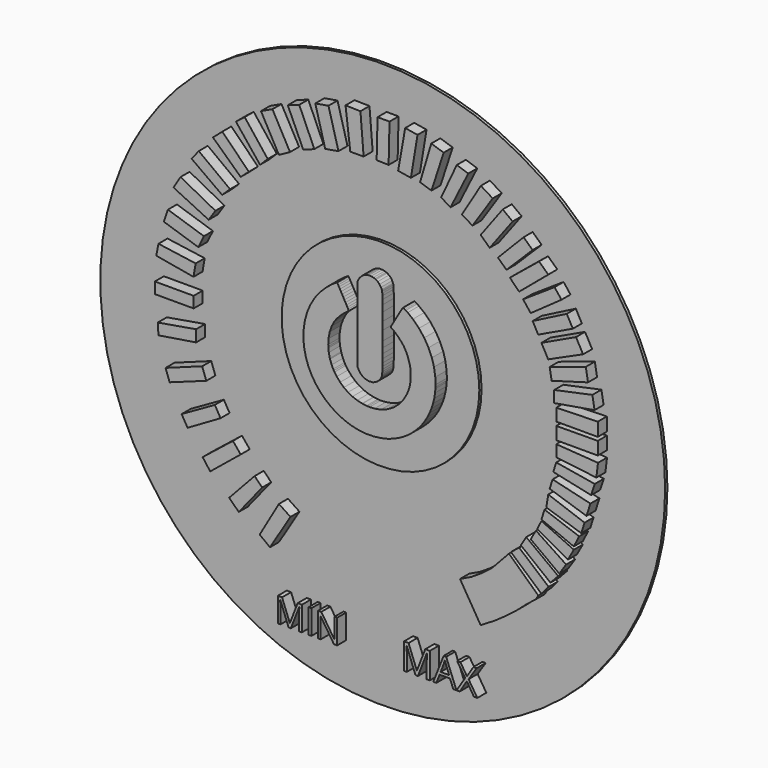
from build123d import *

# Parameters (mm, degrees)
F0_R           = 2.54
F1_DEPTH       = 0.0254
F2_W           = 0.3490758827
F2_H           = 0.1000400152
F2_TEXT_SIZE   = 0.3071047508
F2_TEXT_SIZE_2 = 0.3277752613
F3_DEPTH       = 0.127
F4_R           = 0.889
F5_DEPTH       = 0.0254
F7_DEPTH       = 0.127


# Not quite as in the source:
# - ends of sketch curves that miss each other by under 0.0002 mm in the source are joined
# - Text() gives the source's letters only with a copy of the font that has no kerning and outlines rounded to 1/6400 em; it was checked with that copy


with BuildPart() as f1:
    # F0 (on Front) → F1 (new body)
    with BuildSketch(Plane.XZ):
        Circle(F0_R)
    extrude(amount=F1_DEPTH)


with BuildPart() as f3:
    # F2 (on Front) → F3 (new body)
    with BuildSketch(Plane.XZ):
        Polygon((-0.7486930699, -1.249458408), (-0.8522805874, -1.1806365801), (-1.0253995424, -1.4793376904), (-0.9331640322, -1.550288056), align=None)
        Polygon((-1.0708076879, -1.0309312493), (-1.299977419, -1.2771290494), (-1.2134179706, -1.3615600765), (-1.0026954114, -1.0990436422), align=None)
        Polygon((-1.2657810396, -0.8157898695), (-1.5383707359, -1.0330599034), (-1.470258343, -1.1238763109), (-1.1963900179, -0.9010921931), align=None)
        Polygon((-1.4288047821, -0.5841806325), (-1.7270988319, -0.7535153418), (-1.6738859704, -0.8450413588), (-1.3773700873, -0.6726482062), align=None)
        Polygon((-1.542523179, -0.3150043123), (-1.8718375359, -0.4349482188), (-1.8349434249, -0.537116779), (-1.5053015876, -0.4180797436), align=None)
        Polygon((-1.5972596593, -0.0397546464), (-1.9420784665, -0.0986434607), (-1.9356929697, -0.1979739754), (-1.5972596593, -0.1440516935), align=None)
        with Locations((-1.7937922967, 0.1677751752)):
            Rectangle(F2_W, F2_H)
        Polygon((-1.6008708342, 0.4801122653), (-1.9356929697, 0.5271387636), (-1.9555590115, 0.4263892479), (-1.6206733417, 0.3675004409), align=None)
        Polygon((-1.5271444572, 0.7197599625), (-1.8503724132, 0.8249969687), (-1.8879570998, 0.7175048813), (-1.5775078209, 0.6167780375), align=None)
        Polygon((-1.4236147854, 0.9546708053), (-1.7368667759, 1.1204122566), (-1.8006082597, 1.0164645788), (-1.4842979144, 0.8633332909), align=None)
        Polygon((-1.2918645516, 1.1685207719), (-1.5729977749, 1.3789947843), (-1.6376433196, 1.2970602838), (-1.3632754562, 1.1001166422), align=None)
        Polygon((-1.3615080388, 1.6016833251), (-1.4455363853, 1.5283820685), (-1.1963900179, 1.2964677054), (-1.1228317162, 1.3612192124), align=None)
        Polygon((-1.1603762396, 1.782254898), (-1.2390410993, 1.720574568), (-1.0221891652, 1.4491695712), (-0.9530306811, 1.5178138794), align=None)
        Polygon((-0.9107137304, 1.9256875701), (-1.0137734935, 1.8770102179), (-0.8522805874, 1.5829110052), (-0.7525596556, 1.6376687958), align=None)
        Polygon((-0.6696148776, 2.0388094708), (-0.7724154857, 2.0021589007), (-0.6338581443, 1.6955448082), (-0.5339671768, 1.7319274092), align=None)
        Polygon((-0.4066344177, 2.1170291116), (-0.5253467243, 2.0967551973), (-0.4360276186, 1.7660134806), (-0.3169880365, 1.7863432877), align=None)
        Polygon((-0.1192599157, 2.1669168491), (-0.2532047802, 2.1701059304), (-0.210682585, 1.8171718111), (-0.0905574489, 1.8171718111), align=None)
        Polygon((0.1423002043, 2.1701059304), (0.0346301167, 2.1701059304), (0.0264544585, 1.8267194424), (0.1340635463, 1.8241573872), align=None)
        Polygon((0.2833104756, 2.1649370385), (0.2196951536, 1.8059734721), (0.3347366001, 1.7870105803), (0.3940240595, 2.1466875312), align=None)
        Polygon((0.5177668846, 2.1187307883), (0.4169090826, 1.7794254236), (0.5195422942, 1.7460099602), (0.6290923937, 2.0824852746), align=None)
        Polygon((0.747175936, 2.0229304042), (0.6065378548, 1.720574568), (0.6906718071, 1.668983007), (0.8505268488, 1.9892812707), align=None)
        Polygon((0.9638413755, 1.9291095066), (0.7936382317, 1.6466851812), (0.8879552338, 1.5888492988), (1.07054635, 1.8636772281), align=None)
        Polygon((1.1605156012, 1.8059734721), (0.9617757169, 1.5392288333), (1.0429997554, 1.4636225888), (1.2494549805, 1.739387859), align=None)
        Polygon((1.3480731888, 1.6466851812), (1.1172712548, 1.4102814021), (1.1943845382, 1.3385015957), (1.4289910866, 1.5713639035), align=None)
        Polygon((1.4869238318, 1.5001156922), (1.2247274863, 1.2863905868), (1.3078704694, 1.2026248262), (1.5698518837, 1.4229232911), align=None)
        Polygon((1.6264292635, 1.341770908), (1.3435615692, 1.1536504608), (1.4119567959, 1.0664216649), (1.6886859667, 1.2623709626), align=None)
        Polygon((1.7362208883, 1.1663370695), (1.429526601, 1.0095325997), (1.4795911422, 0.9183586745), (1.7910854658, 1.0664216649), align=None)
        Polygon((1.8194396473, 1.0095325997), (1.5084119514, 0.8625953342), (1.5692590569, 0.7517849818), (1.8830887275, 0.8936194936), align=None)
        Polygon((1.9073629924, 0.8022663837), (1.582456287, 0.6956063444), (1.6001283772, 0.592128814), (1.9272749778, 0.6856733235), align=None)
        Polygon((1.9666856626, 0.5995435624), (1.6236074734, 0.5271387636), (1.6236074734, 0.4231569183), (1.9862328128, 0.485086766), align=None)
        Polygon((2.015253529, 0.4032908764), (1.6420545289, 0.3933578264), (1.6420545289, 0.2826752607), (2.015253529, 0.2826752607), align=None)
        Polygon((2.015253529, 0.251457066), (1.6420545289, 0.2486190933), (1.6420545289, 0.1350984676), (2.015253529, 0.1350984676), align=None)
        Polygon((2.017248075, 0.0780963971), (1.6420545289, 0.1038802948), (1.6420545289, 0), (2.0024825353, -0.0436964438), align=None)
        Polygon((1.9879953374, -0.0986434607), (1.6420545289, -0.0408584456), (1.614824855, -0.1244924462), (1.9556551706, -0.1979739754), align=None)
        Polygon((1.9490479923, -0.266705432), (1.6094174935, -0.1855972077), (1.582456287, -0.2684066297), (1.9134117615, -0.3761595721), align=None)
        Polygon((0.8798243362, -1.1947943131), (0.7763660396, -1.2446495239), (0.9617757169, -1.550288056), (1.0897380215, -1.4726622101), (1.1945230654, -1.3990064617), (1.2936473526, -1.3212840993), (1.3782845344, -1.2471727096), (1.4573722822, -1.1851607973), (1.4806979029, -1.1471220829), (1.2163871784, -0.9010921931), (1.1444232419, -0.9784032881), (1.0681968129, -1.060293593), (0.9777066291, -1.1312460413), align=None)
        Polygon((1.2338161469, -0.8828166756), (1.5084119514, -1.1238763109), (1.5735052293, -1.0481916834), (1.308486416, -0.8242684642), align=None)
        Polygon((1.3227950194, -0.7999772306), (1.5895956894, -1.0097532067), (1.6593816735, -0.9347818932), (1.3720442725, -0.7196630432), align=None)
        Polygon((1.8964227956, -0.4349482188), (1.5699296491, -0.3178600746), (1.5521479478, -0.4257356384), (1.8661382509, -0.5279650368), align=None)
        Polygon((1.5084119514, -0.5357319337), (1.799666672, -0.6548673846), (1.8479382852, -0.5592181114), (1.5368546592, -0.4483721859), align=None)
        Polygon((1.799666672, -0.6807283975), (1.5084119514, -0.5475971848), (1.4707046794, -0.624474138), (1.7460315721, -0.7773342659), align=None)
        Polygon((1.4119567959, -0.7232087664), (1.6691774363, -0.9126354125), (1.7306674636, -0.8200833912), (1.459391008, -0.6398518152), align=None)
        with Locations((-0.8928100578, -2.1302874666)):
            Text('MIN', F2_TEXT_SIZE, font='Open Sans', text_align=(TextAlign.LEFT, TextAlign.BOTTOM))
        with Locations((0.2404058614, -2.1366658621)):
            Text('MAX', F2_TEXT_SIZE_2, font='Open Sans', text_align=(TextAlign.LEFT, TextAlign.BOTTOM))
    extrude(amount=F3_DEPTH)


with BuildPart() as f5:
    # F4 (on face) → F5 (new body)
    with BuildSketch(Plane.XZ.offset(0.0254)):
        with Locations((0, 0.2540000423)):
            Circle(F4_R)
    extrude(amount=F5_DEPTH)


with BuildPart() as f7:
    # F6 (on face) → F7 (new body)
    with BuildSketch(Plane.XZ.offset(0.0508)):
        Polygon((-0.314813559, 0.7605155762), (-0.3176653374, 0.7585868734), (-0.3344407987, 0.7473923925), (-0.3820504885, 0.7096888803), (-0.4384131367, 0.6546145355), (-0.4864580979, 0.5939642135), (-0.5258699254, 0.5283708089), (-0.5563254177, 0.4584747212), (-0.5774973707, 0.3848738231), (-0.58907409, 0.3082185203), (-0.5915849058, 0.2488314861), (-0.590743381, 0.2290966793), (-0.5899698986, 0.2110053974), (-0.58333326, 0.1568666361), (-0.5684265797, 0.0905749263), (-0.5467940776, 0.0292729746), (-0.5167743571, -0.0320052389), (-0.4803316311, -0.0888306757), (-0.4380302517, -0.140838108), (-0.3904330697, -0.1876072736), (-0.3380979331, -0.2287704432), (-0.2815751851, -0.263920363), (-0.2214226735, -0.2926792973), (-0.1581907416, -0.3146519996), (-0.0954341628, -0.3287765888), (-0.0288357049, -0.3358796696), (0.0402448742, -0.3351334542), (0.1101809869, -0.3260402836), (0.1631665291, -0.3136898318), (0.1803872681, -0.3082069126), (0.1915167085, -0.3046509451), (0.2243872068, -0.2922462094), (0.2665560036, -0.2731370428), (0.3067560727, -0.2510425145), (0.3448923547, -0.226110967), (0.3808172578, -0.1985062525), (0.4144182116, -0.1683899717), (0.4455801444, -0.1359247261), (0.4741779782, -0.1012481015), (0.5001016444, -0.064552718), (0.5232135572, -0.0259511458), (0.5434061495, 0.0143539888), (0.5605493401, 0.0562376078), (0.5745255558, 0.0995195987), (0.5852247278, 0.1440598744), (0.5925092705, 0.1896758209), (0.595781311, 0.224582589), (0.5962691152, 0.2362248492), (0.597072116, 0.2558395811), (0.5944930076, 0.3148763969), (0.5828882708, 0.3913265718), (0.5638837732, 0.4581598426), (0.5337950096, 0.5280309148), (0.4950208298, 0.593484232), (0.4479389691, 0.6537718278), (0.3929471758, 0.7081657482), (0.3467333566, 0.7450162285), (0.3304231854, 0.7558980144), (0.3279766597, 0.7574764988), (0.3205945562, 0.7620743661), (0.3120467257, 0.7671525328), (0.3056402306, 0.7706121903), (0.305309257, 0.7707793156), (0.3033294196, 0.7684255089), (0.2979535672, 0.7611684833), (0.2909366914, 0.7504467972), (0.2849804771, 0.7407007195), (0.2830667837, 0.7374036634), (0.280512691, 0.7328283102), (0.2727503503, 0.7191772973), (0.2587316081, 0.6947595702), (0.2428917302, 0.6673449743), (0.2310568499, 0.6469347463), (0.2271218961, 0.6401204969), (0.1927948775, 0.5806231562), (0.2150345045, 0.5648144424), (0.2216010995, 0.5602015657), (0.2401551699, 0.5446593735), (0.2670144196, 0.5191859881), (0.2915922465, 0.4924643243), (0.3057735901, 0.4748633482), (0.3098886563, 0.4685794295), (0.3154521257, 0.4601216551), (0.3303389092, 0.4335075584), (0.3471819126, 0.3961442583), (0.360062445, 0.3574776456), (0.3605971736, 0.355234596), (0.3620810576, 0.350780062), (0.3690303913, 0.3216293834), (0.3706163803, 0.311790748), (0.3719897367, 0.3033755001), (0.3735357008, 0.2776819775), (0.3731804793, 0.2372267493), (0.3698834232, 0.1972167988), (0.3661110708, 0.1724888782), (0.3640222682, 0.1644663753), (0.3597320928, 0.1480311262), (0.3410704552, 0.1002313179), (0.3076846356, 0.0421325871), (0.2645777538, -0.008721626), (0.226388939, -0.0419048193), (0.2125327982, -0.0512831677), (0.2000875372, -0.0596834062), (0.1602001631, -0.08112928), (0.1055185633, -0.1014469502), (0.0479751788, -0.1123037206), (0.0022241481, -0.1145701339), (-0.0129478133, -0.1138221675), (-0.0246075844, -0.113239304), (-0.059431801, -0.108651443), (-0.0617714796, -0.1080933521), (-0.0634999681, -0.1078656352), (-0.108112789, -0.097223999), (-0.1505242371, -0.0812915634), (-0.1903991033, -0.0603084782), (-0.2274071819, -0.034469865), (-0.261228273, -0.0039858549), (-0.2915071551, 0.0309309194), (-0.3119198846, 0.0599365075), (-0.3179061177, 0.0700603208), (-0.323402045, 0.0793861365), (-0.3376134073, 0.1086994164), (-0.3520098851, 0.148982037), (-0.3525864772, 0.1516447197), (-0.3540284976, 0.1556796206), (-0.3632742634, 0.1983762465), (-0.3670866408, 0.2327401761), (-0.3675194107, 0.2442198349), (-0.3681448007, 0.2596669679), (-0.3658908951, 0.3061384478), (-0.3554944118, 0.3631389938), (-0.3359122002, 0.4168950165), (-0.3149166072, 0.4565772626), (-0.3067189951, 0.4690100158), (-0.302443829, 0.4754715452), (-0.2877171454, 0.4935628271), (-0.2622562678, 0.5210049402), (-0.2347090891, 0.546953622), (-0.2160574578, 0.5624407799), (-0.2094358285, 0.5670011238), (-0.2068442124, 0.5687897392), (-0.1990393452, 0.5741380744), (-0.1903264118, 0.5800692732), (-0.1842326116, 0.5842493799), (-0.1824090518, 0.5855198311), (-0.1837874803, 0.5882734825), (-0.1889982298, 0.5981821616), (-0.1958675135, 0.6109676347), (-0.2040776334, 0.6260570446), (-0.213295882, 0.6428725309), (-0.223199558, 0.6608412363), (-0.2334734648, 0.679382799), (-0.2438174154, 0.6979218601), (-0.2538736866, 0.7158630483), (-0.2633320849, 0.7326360081), (-0.2718699092, 0.7476753867), (-0.2791844706, 0.7603908162), (-0.2849405601, 0.7702194454), (-0.2888079719, 0.7765558968), (-0.2889715187, 0.7768622006), (-0.2894752579, 0.7765305632), (-0.2964245915, 0.7723629643), (-0.3061831771, 0.7661891142), align=None)
    extrude(amount=F7_DEPTH)


with BuildPart() as f7b:
    # F6 (on face) → F7, piece 2 (new body)
    with BuildSketch(Plane.XZ.offset(0.0508)):
        Polygon((-0.0164124738, 0.9254409249), (-0.0206050884, 0.9243277307), (-0.0269015149, 0.9226992151), (-0.0450753482, 0.9150444416), (-0.0662460504, 0.9008355808), (-0.0839721045, 0.8818762576), (-0.0951565793, 0.8644904157), (-0.0980708967, 0.8583165656), (-0.1071115345, 0.8388519273), (-0.1071115345, 0.1752430958), (-0.0980708967, 0.156133679), (-0.0958995426, 0.1514132353), (-0.0880821676, 0.137787238), (-0.0764524152, 0.1229229686), (-0.0626087822, 0.1108604463), (-0.0502885993, 0.1030705885), (-0.0459558973, 0.1008992344), (-0.0391041245, 0.0975171253), (-0.0064487604, 0.088519014), (0.0265593237, 0.0897672924), (0.0336012151, 0.0915033751), (0.040372938, 0.0932419593), (0.0707743966, 0.1083613878), (0.094916952, 0.1311230822), (0.0985692296, 0.1366715423), (0.099544838, 0.1381374564), (0.1025342022, 0.1424801646), (0.1059938597, 0.1477759671), (0.1089632114, 0.1531743335), (0.1115173041, 0.159283143), (0.1136486333, 0.1666802559), (0.1154122331, 0.17600357), (0.11685063, 0.1878384504), (0.117976332, 0.2027827697), (0.1188468749, 0.2214569151), (0.1194847727, 0.2444462514), (0.119932552, 0.2723761687), (0.120205222, 0.3058320321), (0.1203678234, 0.3454192189), (0.120432864, 0.3917531131), (0.1204603811, 0.445434089), (0.1204603811, 0.4916429051), (0.1204603811, 0.5070475116), (0.1204603811, 0.5306347207), (0.1204203562, 0.6013713326), (0.1202702626, 0.6757051878), (0.1199725769, 0.7325981667), (0.1194997821, 0.7745768449), (0.1187943422, 0.8041878105), (0.1178137306, 0.8239501345), (0.1165254272, 0.8363953954), (0.1154547596, 0.8422040177), (0.1148944101, 0.8440626768), (0.1131208041, 0.8500088849), (0.1057512084, 0.8672171161), (0.0931008195, 0.8864616171), (0.0763929003, 0.9023140028), (0.0606906082, 0.9125478847), (0.0551396466, 0.9152895944), (0.0510145742, 0.9173233627), (0.0377287891, 0.921545996), (0.0172610252, 0.9254134077), (-0.0032067386, 0.926486577), align=None)
    extrude(amount=F7_DEPTH)


solid = Compound([f1.part, f3.part, f5.part, f7.part, f7b.part])
